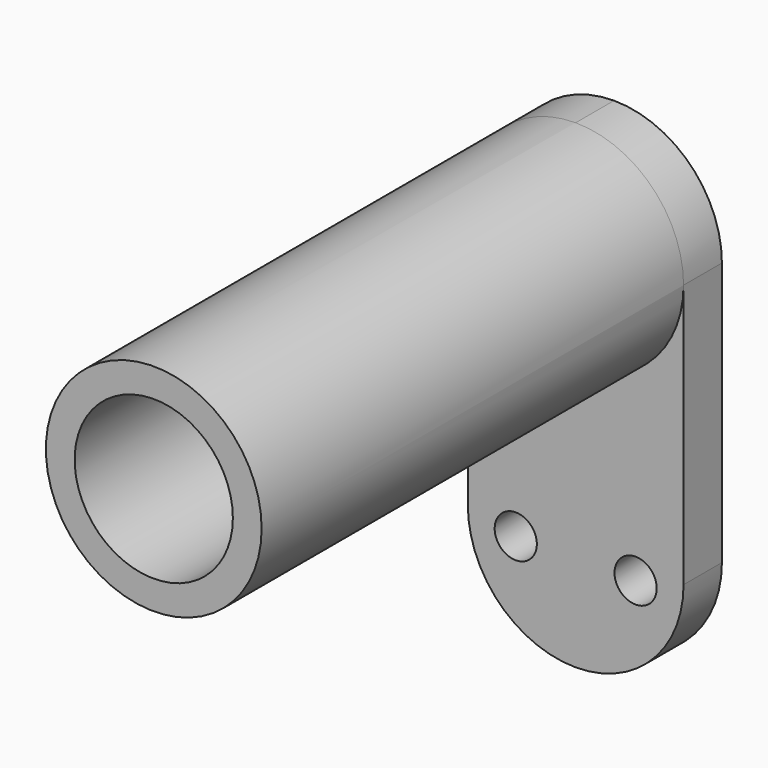
from build123d import *

# Parameters (mm, degrees)
F0_W     = 22.5
F0_H     = 50
F1_DEPTH = 5
F2_D     = 4.4
F4_R     = 11.24999
F3_R     = 11.25
F3_R_2   = 8.25
F5_DEPTH = 55


# Not quite as in the source:
# - a fillet or chamfer is up to 0.001 mm smaller than in the source, because OpenCascade refuses the exact size


with BuildPart() as f1:
    # F0 (on Front) → F1 (new body)
    with BuildSketch(Plane.XZ):
        with Locations((11.25, 25)):
            Rectangle(F0_W, F0_H)
    extrude(amount=F1_DEPTH)

    # F2 (through all)
    with Locations(Plane(origin=(0, 0, 0), x_dir=(1, 0, 0), z_dir=(0, 1, 0))):
        with Locations((5, -10), (17.5, -10)):
            Hole(F2_D / 2)

    # F4 (radius 11.25 in the source; OpenCascade refuses exactly that, so slightly less here)
    f4_edges = [f1.edges().sort_by_distance(p)[0] for p in [
        (22.5, -2.5, 50),
        (0, -2.5, 50),
        (22.5, -2.5, 0),
        (0, -2.5, 0),
    ]]
    fillet(f4_edges, radius=F4_R)

    # F3 (on face) → F5 (join)
    with BuildSketch(Plane.XZ.offset(5)):
        with Locations((11.25, 38.75)):
            Circle(F3_R)
        with Locations((11.25, 38.75)):
            Circle(F3_R_2, mode=Mode.SUBTRACT)
    extrude(amount=F5_DEPTH)


solid = f1.part
